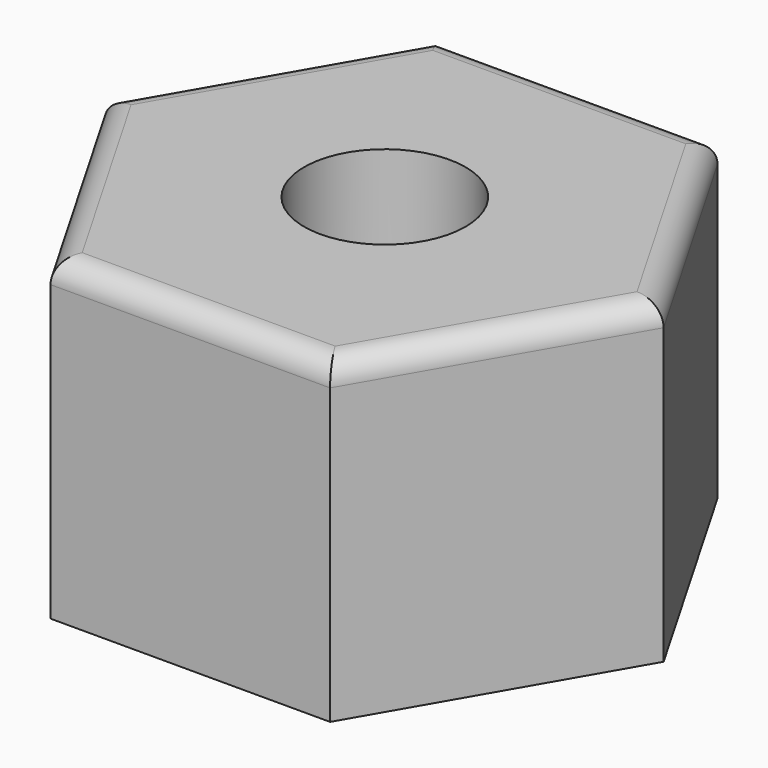
from build123d import *

# Parameters (mm, degrees)
F0_R         = 2.8
F1_DEPTH     = 11
F3_DEPTH     = 2
F5_DEPTH     = 0.5
F6_DEPTH     = 0.5
F7_R         = 0.8
F8_T4_DEPTH  = 7.176254213
F8_S5_R      = 2.8
F8_T6_DEPTH  = 5
F8_T10_DEPTH = 7.240123034
F8_S11_R     = 2.8
F8_T12_DEPTH = 5
F8_T16_DEPTH = 10.9265531961
F8_S17_R     = 2.8
F8_T18_DEPTH = 7
F8_T24_DEPTH = 10.862684375
F8_S25_R     = 2.8
F8_T26_DEPTH = 7
F9_R         = 0.8


# Not quite as in the source:
# - a fillet or chamfer that OpenCascade refuses, or shapes differently, is made with other operations: its cross-section is extruded or revolved along the edge and cut away or added


with BuildPart() as f1:
    # F0 (on Top) → F1 (new body)
    with BuildSketch(Plane.XY):
        Polygon((4.8497422612, -8.4), (9.6994845224, 0), (4.8497422612, 8.4), (-4.8497422612, 8.4), (-9.6994845224, 0), (-4.8497422612, -8.4), align=None)
        with Locations((-0.031784919, 0.0747148006)):
            Circle(F0_R, mode=Mode.SUBTRACT)
    extrude(amount=F1_DEPTH)

    # F2 (on Top) → F3 (cut)
    with BuildSketch(Plane.XY):
        with BuildLine():
            Line((-6, 1.1), (-6, -1.1))
            Line((-6, -1.1), (-3.585038354, -1.1))
            ThreePointArc((-3.585038354, -1.1), (-3.75, 0), (-3.585038354, 1.1))
            Line((-3.585038354, 1.1), (-6, 1.1))
        make_face()
        with BuildLine():
            ThreePointArc((-3.585038354, 1.1), (-3.75, 0), (-3.585038354, -1.1))
            Line((-3.585038354, -1.1), (3.585038354, -1.1))
            ThreePointArc((3.585038354, -1.1), (3.7085302903, -0.556150237), (3.75, 0))
            ThreePointArc((3.75, 0), (3.7085302903, 0.556150237), (3.585038354, 1.1))
            Line((3.585038354, 1.1), (-3.585038354, 1.1))
        make_face()
        with BuildLine():
            ThreePointArc((3.75, 0), (3.7085302903, -0.556150237), (3.585038354, -1.1))
            Line((3.585038354, -1.1), (6, -1.1))
            Line((6, -1.1), (6, 1.1))
            Line((6, 1.1), (3.585038354, 1.1))
            ThreePointArc((3.585038354, 1.1), (3.7085302903, 0.556150237), (3.75, 0))
        make_face()
    extrude(amount=F3_DEPTH, mode=Mode.SUBTRACT)

    # F4 (on face) → F5 (join)
    with BuildSketch(Plane(origin=(0, 0, 0), x_dir=(1, 0, 0), z_dir=(0, 0, -1))):
        with BuildLine():
            Line((2.509876966, 1.1), (3.585038354, 1.1))
            ThreePointArc((3.585038354, 1.1), (0, 3.75), (-3.585038354, 1.1))
            Line((-3.585038354, 1.1), (-2.5734468039, 1.1))
            ThreePointArc((-2.5734468039, 1.1), (-0.031784919, 2.7252851994), (2.509876966, 1.1))
        make_face()
    extrude(amount=F5_DEPTH)

    # F4 (on face) → F6 (join)
    with BuildSketch(Plane(origin=(0, 0, 0), x_dir=(1, 0, 0), z_dir=(0, 0, -1))):
        with BuildLine():
            ThreePointArc((-3.585038354, -1.1), (0, -3.75), (3.585038354, -1.1))
            Line((3.585038354, -1.1), (2.573745787, -1.1))
            ThreePointArc((2.573745787, -1.1), (-0.031784919, -2.8747148006), (-2.637315625, -1.1))
            Line((-2.637315625, -1.1), (-3.585038354, -1.1))
        make_face()
    extrude(amount=F6_DEPTH)

    # F7
    f7_edges = [f1.edges().sort_by_distance(p)[0] for p in [
        (-0.031785, 2.874715, -0.5),
        (-0.031785, -2.725285, -0.5),
    ]]
    fillet(f7_edges, radius=F7_R)

    # F8: fillet of radius 1.5 on 4 edges, made by hand


with BuildPart() as f8_tool2:
    # F8_s3 → F8_t4 (new body)
    with BuildSketch(Plane.YZ.offset(6)):
        with BuildLine():
            ThreePointArc((1.1, 0.5), (0.6606601718, 1.5606601718), (-0.4, 2))
            Line((-0.4, 2), (1.1, 2))
            Line((1.1, 2), (1.1, 0.5))
        make_face()
    extrude(amount=-F8_T4_DEPTH)

    # F8_s5 → F8_t6 (cut, symmetric)
    with BuildSketch(Plane.XY.offset(1.2)):
        with Locations((-0.031784919, 0.0747148006)):
            Circle(F8_S5_R)
    extrude(amount=F8_T6_DEPTH, both=True, mode=Mode.SUBTRACT)


with BuildPart() as f1_1:
    add(f1.part)

    # F8_t1: union F8_tool2
    add(f8_tool2.part)


with BuildPart() as f8_tool8:
    # F8_s9 → F8_t10 (new body)
    with BuildSketch(Plane.YZ.offset(-1.240123034)):
        with BuildLine():
            ThreePointArc((0.4, 2), (-0.6606601718, 1.5606601718), (-1.1, 0.5))
            Line((-1.1, 0.5), (-1.1, 2))
            Line((-1.1, 2), (0.4, 2))
        make_face()
    extrude(amount=F8_T10_DEPTH)

    # F8_s11 → F8_t12 (cut, symmetric)
    with BuildSketch(Plane.XY.offset(1.2)):
        with Locations((-0.031784919, 0.0747148006)):
            Circle(F8_S11_R)
    extrude(amount=F8_T12_DEPTH, both=True, mode=Mode.SUBTRACT)


with BuildPart() as f1_2:
    add(f1_1.part)

    # F8_t7: union F8_tool8
    add(f8_tool8.part)


with BuildPart() as f8_tool14:
    # F8_s15 → F8_t16 (new body)
    with BuildSketch(Plane.YZ.offset(-9.75)):
        with BuildLine():
            ThreePointArc((0.4, 2), (-0.6606601718, 1.5606601718), (-1.1, 0.5))
            Line((-1.1, 0.5), (-1.1, 2))
            Line((-1.1, 2), (0.4, 2))
        make_face()
    extrude(amount=F8_T16_DEPTH)

    # F8_s17 → F8_t18 (cut, symmetric)
    with BuildSketch(Plane.XY.offset(1.2)):
        with Locations((-0.031784919, 0.0747148006)):
            Circle(F8_S17_R)
    extrude(amount=F8_T18_DEPTH, both=True, mode=Mode.SUBTRACT)

    split(bisect_by=Plane(origin=(-7.2746133918, -4.2, 0), x_dir=(0, 0, 1), z_dir=(0.8660254038, 0.5, 0)), keep=Keep.TOP)

    split(bisect_by=Plane(origin=(-7.2746133918, 4.2, 0), x_dir=(0, 0, 1), z_dir=(0.8660254038, -0.5, 0)), keep=Keep.TOP)


with BuildPart() as f1_3:
    add(f1_2.part)

    # F8_t13: union F8_tool14
    add(f8_tool14.part)


with BuildPart() as f8_tool22:
    # F8_s23 → F8_t24 (new body)
    with BuildSketch(Plane.YZ.offset(1.112684375)):
        with BuildLine():
            ThreePointArc((1.1, 0.5), (0.6606601718, 1.5606601718), (-0.4, 2))
            Line((-0.4, 2), (1.1, 2))
            Line((1.1, 2), (1.1, 0.5))
        make_face()
    extrude(amount=-F8_T24_DEPTH)

    # F8_s25 → F8_t26 (cut, symmetric)
    with BuildSketch(Plane.XY.offset(1.2)):
        with Locations((-0.031784919, 0.0747148006)):
            Circle(F8_S25_R)
    extrude(amount=F8_T26_DEPTH, both=True, mode=Mode.SUBTRACT)

    split(bisect_by=Plane(origin=(-7.2746133918, -4.2, 0), x_dir=(0, 0, 1), z_dir=(0.8660254038, 0.5, 0)), keep=Keep.TOP)

    split(bisect_by=Plane(origin=(-7.2746133918, 4.2, 0), x_dir=(0, 0, 1), z_dir=(0.8660254038, -0.5, 0)), keep=Keep.TOP)


with BuildPart() as f1_4:
    add(f1_3.part)

    # F8_t21: union F8_tool22
    add(f8_tool22.part)

    # F9
    f9_edges = [f1_4.edges().sort_by_distance(p)[0] for p in [
        (0, -8.4, 11),
        (7.274613, -4.2, 11),
        (7.274613, 4.2, 11),
        (0, 8.4, 11),
        (-7.274613, 4.2, 11),
        (-7.274613, -4.2, 11),
    ]]
    fillet(f9_edges, radius=F9_R)


solid = f1_4.part
